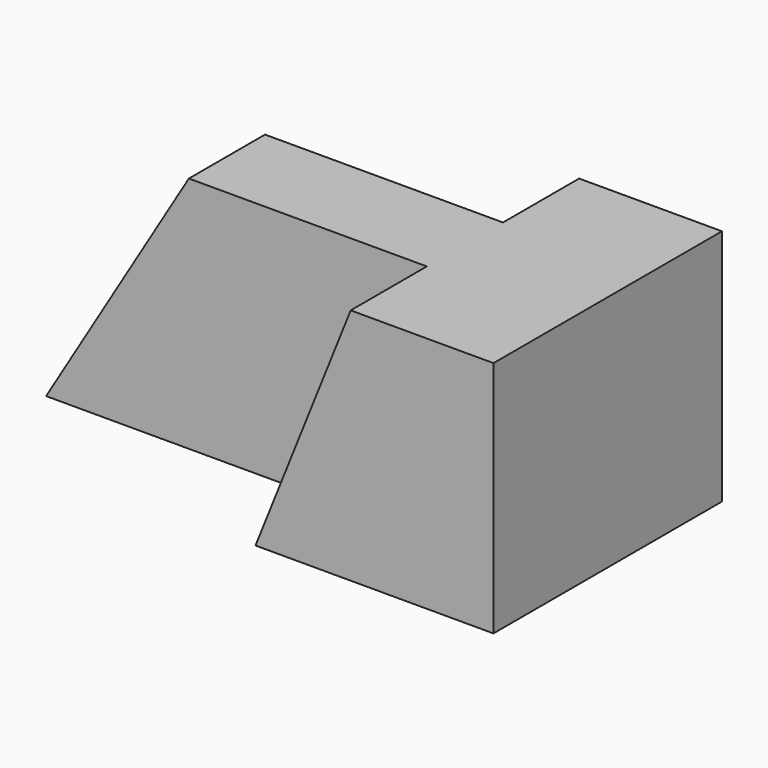
from build123d import *

# Parameters (mm, degrees)
F0_W     = 69.85
F0_H     = 31.75
F1_DEPTH = 38.1
F3_DEPTH = 12.7
F5_DEPTH = 12.7
F7_DEPTH = 25.401


# Not quite as in the source:
# - a feature names something its author has since deleted; it is built from what else it names


with BuildPart() as f1:
    # F0 (on Front) → F1 (new body)
    with BuildSketch(Plane.XZ):
        with Locations((-34.925, 15.875)):
            Rectangle(F0_W, F0_H)
    extrude(amount=F1_DEPTH)

    # F2 (on face) → F3 (cut)
    with BuildSketch(Plane(origin=(0, 0, 0), x_dir=(-1, 0, 0), z_dir=(0, 1, 0))):
        Polygon((69.85, 31.75), (19.05, 31.75), (31.75, 0), (69.85, 0), align=None)
    extrude(amount=-F3_DEPTH, mode=Mode.SUBTRACT)

    # F4 (on face) → F5 (cut)
    with BuildSketch(Plane.XZ.offset(38.1)):
        Polygon((-31.75, 0), (-19.05, 31.75), (-69.85, 31.75), (-69.85, 0), align=None)
    extrude(amount=-F5_DEPTH, mode=Mode.SUBTRACT)

    # F6 (on face) → F7 (cut, through all)
    with BuildSketch(Plane.XZ.offset(25.4)):
        Polygon((-69.85, 0), (-50.8, 31.75), (-69.85, 31.75), align=None)
    extrude(amount=-F7_DEPTH, mode=Mode.SUBTRACT)


solid = f1.part
